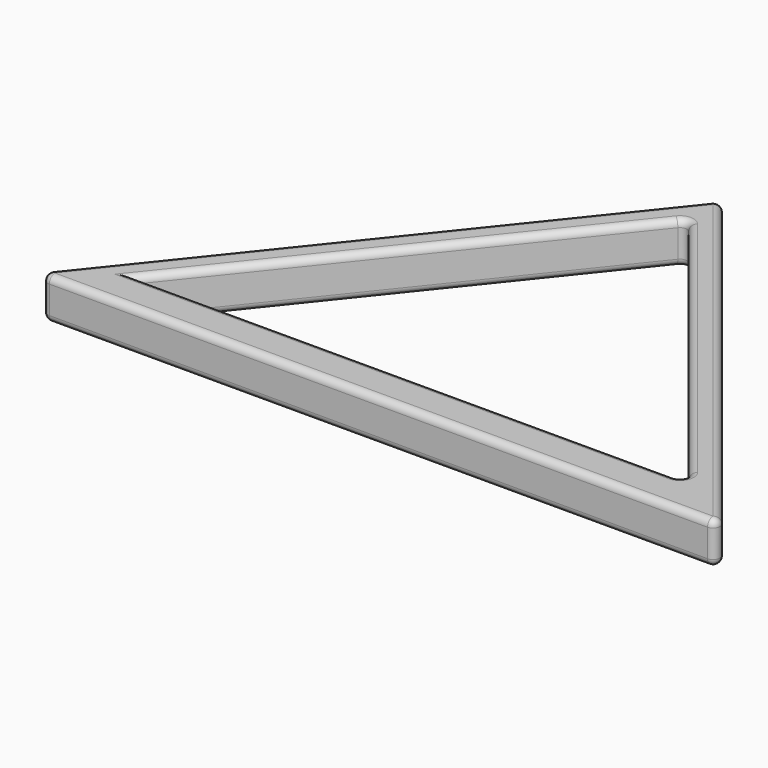
from build123d import *

# Parameters (mm, degrees)
F1_DEPTH = 30
F2_R     = 5


with BuildPart() as f1:
    # F0 (on Top) → F1 (new body)
    with BuildSketch(Plane.XY):
        Polygon((-248, -30), (0, -30), (248, -30), (0, 280), align=None)
        Polygon((200, 0), (0, 0), (-200, 0), (0, 250), align=None, mode=Mode.SUBTRACT)
    extrude(amount=F1_DEPTH)

    # F2
    f2_edges = [f1.edges().sort_by_distance(p)[0] for p in [
        (0, 280, 15),
        (-248, -30, 15),
        (-124, 125, 0),
        (-124, 125, 30),
        (248, -30, 15),
        (124, 125, 0),
        (124, 125, 30),
        (0, -30, 30),
        (0, -30, 0),
        (0, 0, 30),
        (-100, 125, 30),
        (0, 250, 15),
        (200, 0, 15),
        (100, 125, 0),
        (100, 125, 30),
        (0, 0, 0),
        (-100, 125, 0),
    ]]
    fillet(f2_edges, radius=F2_R)


solid = f1.part
